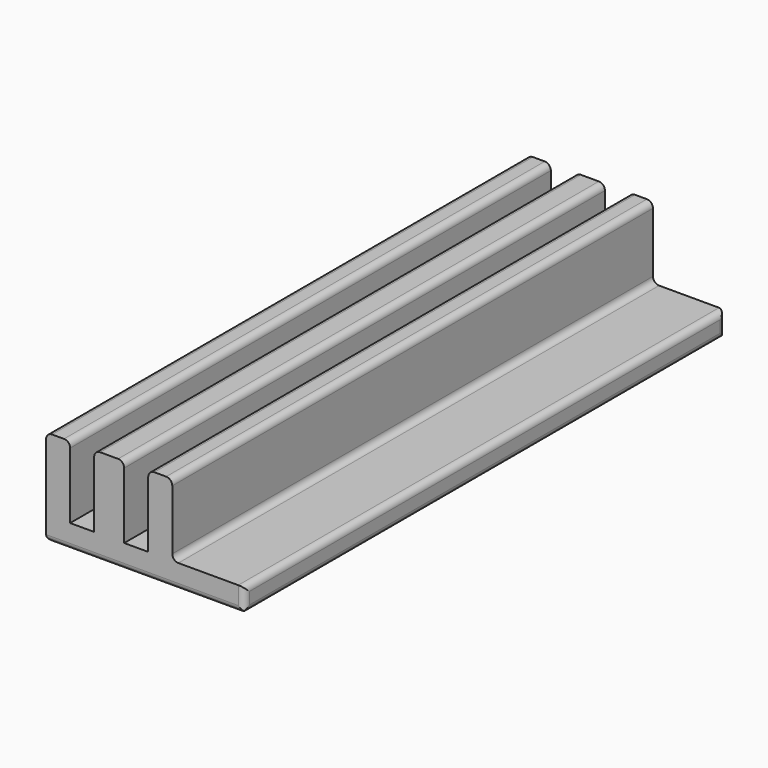
from build123d import *

# Parameters (mm, degrees)
F1_DEPTH    = 50
F2_T1_DEPTH = 52.54
F2_T3_DEPTH = 4.54
F3_R        = 0.508
F4_T1_DEPTH = 18.532
F4_T3_DEPTH = 52.54
F5_R        = 0.508


# Not quite as in the source:
# - a fillet or chamfer that OpenCascade refuses, or shapes differently, is made with other operations: its cross-section is extruded or revolved along the edge and cut away or added


with BuildPart() as f1:
    # F0 (on Front) → F1 (new body)
    with BuildSketch(Plane.XZ):
        Polygon((0, 8), (0, 0), (16.5, 0), (16.5, 2), (10.5, 2), (10.5, 8), (8.5, 8), (8.5, 2), (6.5, 2), (6.5, 8), (4, 8), (4, 2), (2, 2), (2, 8), align=None)
    extrude(amount=F1_DEPTH)

    # F2: fillet of radius 0.508 on 4 edges, made by hand

    # F2_s2 → F2_t1 (cut)
    with BuildSketch(Plane.XZ.offset(-1.27)):
        with BuildLine():
            ThreePointArc((15.992, 0), (16.3512102448, 0.1487897552), (16.5, 0.508))
            Line((16.5, 0.508), (16.5, 0))
            Line((16.5, 0), (15.992, 0))
        make_face()
        with BuildLine():
            ThreePointArc((16.5, 1.492), (16.3512102448, 1.8512102448), (15.992, 2))
            Line((15.992, 2), (16.5, 2))
            Line((16.5, 2), (16.5, 1.492))
        make_face()
    extrude(amount=F2_T1_DEPTH, mode=Mode.SUBTRACT)

    # F2_s4 → F2_t3 (cut)
    with BuildSketch(Plane.XY.offset(-1.27)):
        with BuildLine():
            ThreePointArc((16.5, -0.508), (16.3512102448, -0.1487897552), (15.992, 0))
            Line((15.992, 0), (16.5, 0))
            Line((16.5, 0), (16.5, -0.508))
        make_face()
        with BuildLine():
            ThreePointArc((16.5, -49.492), (16.3512102448, -49.8512102448), (15.992, -50))
            Line((15.992, -50), (16.5, -50))
            Line((16.5, -50), (16.5, -49.492))
        make_face()
    extrude(amount=F2_T3_DEPTH, mode=Mode.SUBTRACT)

    # F3
    f3_edges = [f1.edges().sort_by_distance(p)[0] for p in [
        (8.5, -25, 8),
        (10.5, -25, 8),
        (6.5, -25, 8),
        (4, -25, 8),
        (2, -25, 8),
        (0, -25, 8),
    ]]
    fillet(f3_edges, radius=F3_R)

    # F4: fillet of radius 0.508 on 4 edges, made by hand

    # F4_s2 → F4_t1 (cut)
    with BuildSketch(Plane.YZ.offset(-1.27)):
        with BuildLine():
            ThreePointArc((0, 0.508), (-0.1487897552, 0.1487897552), (-0.508, 0))
            Line((-0.508, 0), (0, 0))
            Line((0, 0), (0, 0.508))
        make_face()
        with BuildLine():
            ThreePointArc((-49.492, 0), (-49.8512102448, 0.1487897552), (-50, 0.508))
            Line((-50, 0.508), (-50, 0))
            Line((-50, 0), (-49.492, 0))
        make_face()
    extrude(amount=F4_T1_DEPTH, mode=Mode.SUBTRACT)

    # F4_s4 → F4_t3 (cut)
    with BuildSketch(Plane.XZ.offset(-1.27)):
        with BuildLine():
            ThreePointArc((0, 0.508), (0.1487897552, 0.1487897552), (0.508, 0))
            Line((0.508, 0), (0, 0))
            Line((0, 0), (0, 0.508))
        make_face()
    extrude(amount=F4_T3_DEPTH, mode=Mode.SUBTRACT)

    # F5
    f5_edges = [f1.edges().sort_by_distance(p)[0] for p in [
        (10.5, -25, 2),
    ]]
    fillet(f5_edges, radius=F5_R)


solid = f1.part
